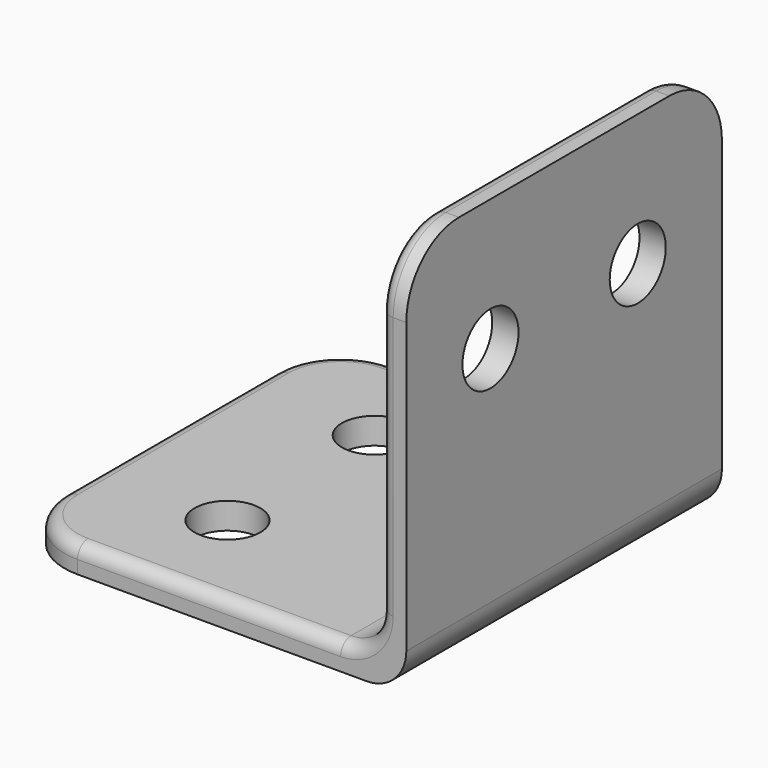
from build123d import *

# Parameters (mm, degrees)
F1_DEPTH = 15
F2_R     = 3
F3_R     = 2.5
F4_DEPTH = 2.001
F5_R     = 5
F6_R     = 1
F7_R     = 2.6650989984
F8_DEPTH = 2.001


# Not quite as in the source:
# - a pattern or mirror of a feature is missing from the dataset's text; its kind, count and spacing are read off the source's solid


with BuildPart() as f1:
    # F0 (on Front) → F1 (new body, symmetric)
    with BuildSketch(Plane.XZ):
        Polygon((-30, 2), (-30, 0), (0, 0), (0, 30), (-2, 30), (-2, 2), align=None)
    extrude(amount=F1_DEPTH, both=True)

    # F2
    f2_edges = [f1.edges().sort_by_distance(p)[0] for p in [
        (0, 0, 0),
        (-2, 0, 2),
    ]]
    fillet(f2_edges, radius=F2_R)

    # F3 (on face) → F4 (cut, through all)
    with BuildSketch(Plane.XY.offset(2)):
        with Locations((-20, 7)):
            Circle(F3_R)
        with Locations((-20, -7)):
            Circle(F3_R)
    extrude(amount=-F4_DEPTH, mode=Mode.SUBTRACT)

    # F5
    f5_edges = [f1.edges().sort_by_distance(p)[0] for p in [
        (-30, -15, 1),
        (-30, 15, 1),
        (-1, -15, 30),
        (-1, 15, 30),
    ]]
    fillet(f5_edges, radius=F5_R)

    # F6
    f6_edges = [f1.edges().sort_by_distance(p)[0] for p in [
        (-15, 15, 2),
        (-28.535534, 13.535534, 2),
        (-30, 0, 2),
        (-15, -15, 2),
        (-28.535534, -13.535534, 2),
        (-2.87868, 15, 2.87868),
        (-2, 15, 15),
        (-2.87868, -15, 2.87868),
        (-2, -15, 15),
        (-2, 13.535534, 28.535534),
        (-2, 0, 30),
        (-2, -13.535534, 28.535534),
    ]]
    fillet(f6_edges, radius=F6_R)

    # F7 (on face) → F8 (cut, through all)
    with BuildSketch(Plane(origin=(-2, 0, 0), x_dir=(0, -1, 0), z_dir=(-1, 0, 0))):
        with Locations((-7, 20)):
            Circle(F7_R)
    f8 = extrude(amount=-F8_DEPTH, mode=Mode.SUBTRACT)

    # F8_copies: F8 across plane
    add(f8.mirror(Plane(origin=(0, 0, 0), x_dir=(0, 0, -1), z_dir=(0, -1, 0))), mode=Mode.SUBTRACT)


solid = f1.part
